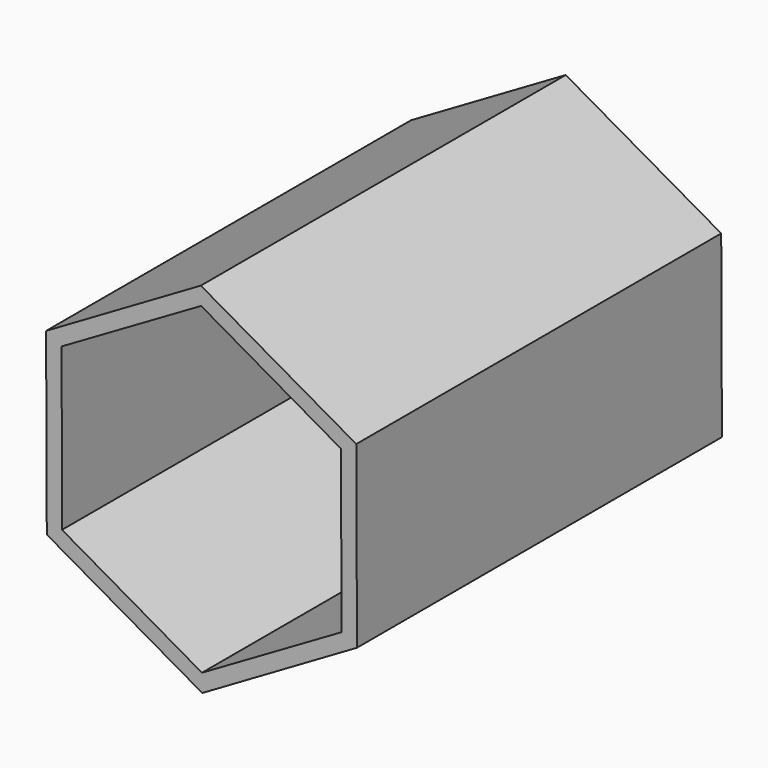
from build123d import *

# Parameters (mm, degrees)
F1_DEPTH = 165.1
F2_DEPTH = 127
F4_DEPTH = 146.05


# Not quite as in the source:
# - a feature names something its author has since deleted; it is built from what else it names


with BuildPart() as f1:
    # F0 (on Front) → F1 (new body)
    with BuildSketch(Plane.XZ):
        Polygon((-0.2583676879, 64.8191452859), (-56.2642103132, 32.1858196618), (-56.0058426253, -32.6333256242), (0.2583676879, -64.8191452859), (56.2642103132, -32.1858196618), (56.0058426253, 32.6333256242), align=None)
    extrude(amount=F1_DEPTH)

    # F0 (on Front) → F2 (join)
    with BuildSketch(Plane.XZ):
        Polygon((-0.2583676879, 64.8191452859), (-56.2642103132, 32.1858196618), (-56.0058426253, -32.6333256242), (0.2583676879, -64.8191452859), (56.2642103132, -32.1858196618), (56.0058426253, 32.6333256242), align=None)
    extrude(amount=F2_DEPTH)

    # F3 (on face) → F4 (cut)
    with BuildSketch(Plane.XZ.offset(165.1)):
        Polygon((-0.1502408993, 58.3915630752), (-50.6436974394, 29.0656691021), (-50.4934565401, -29.3258939731), (0.1502408993, -58.3915630752), (50.6436974394, -29.0656691021), (50.4934565401, 29.3258939731), align=None)
    extrude(amount=-F4_DEPTH, mode=Mode.SUBTRACT)


solid = f1.part
